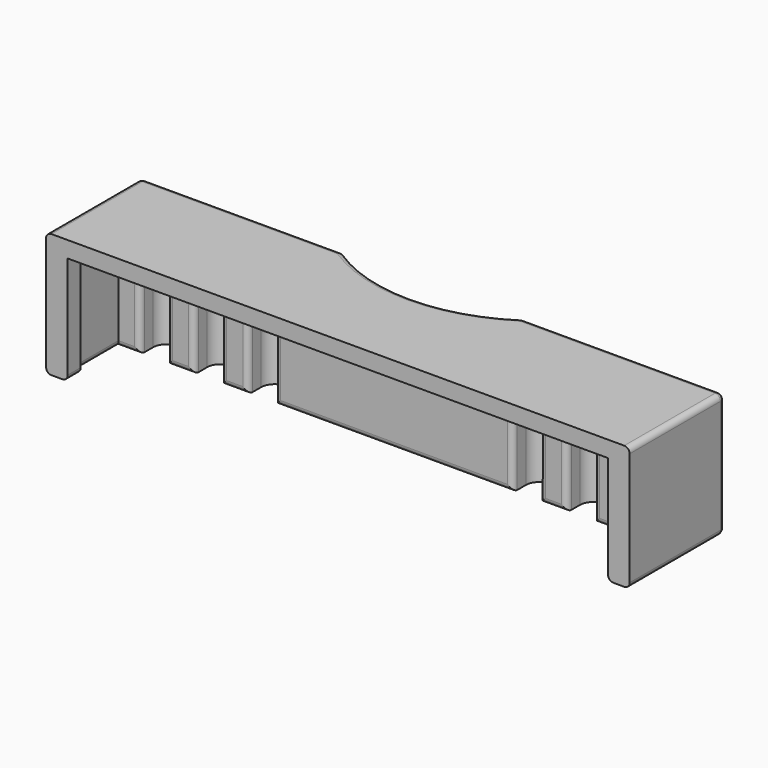
from build123d import *

# Parameters (mm, degrees)
F0_W     = 1
F0_H     = 20
F0_W_2   = 100
F1_DEPTH = 22
F2_DEPTH = 13
F3_DEPTH = 3
F5_DEPTH = 23
F4_W     = 5
F4_H     = 3
F6_DEPTH = 20
F7_R     = 0.9999


# Not quite as in the source:
# - a fillet or chamfer is up to 0.001 mm smaller than in the source, because OpenCascade refuses the exact size
# - a feature names something its author has since deleted; it is built from what else it names


with BuildPart() as f1:
    # F0 (on Front) → F1 (new body)
    with BuildSketch(Plane.XZ):
        Polygon((51, 20), (51, 0), (54, 0), (54, 23), (-54, 23), (-54, 0), (-51, 0), (-51, 20), (-50, 20), (50, 20), align=None)
        with Locations((-50.5, 10)):
            Rectangle(F0_W, F0_H)
        with Locations((0, 10)):
            Rectangle(F0_W_2, F0_H)
        with Locations((50.5, 10)):
            Rectangle(F0_W, F0_H)
    extrude(amount=-F1_DEPTH)

    # F0 (on Front) → F2 (cut)
    with BuildSketch(Plane.XZ):
        with Locations((-50.5, 10)):
            Rectangle(F0_W, F0_H)
        with Locations((0, 10)):
            Rectangle(F0_W_2, F0_H)
        with Locations((50.5, 10)):
            Rectangle(F0_W, F0_H)
    extrude(amount=-F2_DEPTH, mode=Mode.SUBTRACT)

    # F0 (on Front) → F3 (join)
    with BuildSketch(Plane.XZ):
        with Locations((-50.5, 10)):
            Rectangle(F0_W, F0_H)
        with Locations((50.5, 10)):
            Rectangle(F0_W, F0_H)
    extrude(amount=-F3_DEPTH)

    # F4 (on face) → F5 (cut, through all)
    with BuildSketch(Plane(origin=(0, 0, 0), x_dir=(1, 0, 0), z_dir=(0, 0, -1))):
        with BuildLine():
            Line((-16.5831239518, -22), (16.5831239518, -22))
            ThreePointArc((16.5831239518, -22), (0, -17), (-16.5831239518, -22))
        make_face()
    extrude(amount=-F5_DEPTH, mode=Mode.SUBTRACT)

    # F4 (on face) → F6 (cut, through all)
    with BuildSketch(Plane(origin=(0, 0, 0), x_dir=(1, 0, 0), z_dir=(0, 0, -1))):
        with Locations((-44.5, -14.5)):
            Rectangle(F4_W, F4_H)
        with Locations((-34.5, -14.5)):
            Rectangle(F4_W, F4_H)
        with Locations((-24.5, -14.5)):
            Rectangle(F4_W, F4_H)
        with Locations((24.5, -14.5)):
            Rectangle(F4_W, F4_H)
        with Locations((34.5, -14.5)):
            Rectangle(F4_W, F4_H)
        with Locations((44.5, -14.5)):
            Rectangle(F4_W, F4_H)
        with BuildLine():
            Line((-42, -16), (-47, -16))
            ThreePointArc((-47, -16), (-44.5, -18.5), (-42, -16))
        make_face()
        with BuildLine():
            Line((-32, -16), (-37, -16))
            ThreePointArc((-37, -16), (-34.5, -18.5), (-32, -16))
        make_face()
        with BuildLine():
            Line((-22, -16), (-27, -16))
            ThreePointArc((-27, -16), (-24.5, -18.5), (-22, -16))
        make_face()
        with BuildLine():
            ThreePointArc((22, -16), (24.5, -18.5), (27, -16))
            Line((27, -16), (22, -16))
        make_face()
        with BuildLine():
            ThreePointArc((32, -16), (34.5, -18.5), (37, -16))
            Line((37, -16), (32, -16))
        make_face()
        with BuildLine():
            ThreePointArc((42, -16), (44.5, -18.5), (47, -16))
            Line((47, -16), (42, -16))
        make_face()
    extrude(amount=-F6_DEPTH, mode=Mode.SUBTRACT)

    # F7 (radius 1 in the source; OpenCascade refuses exactly that, so slightly less here)
    f7_edges = [f1.edges().sort_by_distance(p)[0] for p in [
        (-54, 22, 11.5),
        (54, 22, 11.5),
        (35.291562, 22, 0),
        (-35.291562, 22, 0),
        (54, 11, 0),
        (-54, 11, 0),
        (-54, 11, 23),
        (-35.291562, 22, 23),
        (35.291562, 22, 23),
        (54, 11, 23),
        (-49, 13, 0),
        (-39.5, 13, 0),
        (-29.5, 13, 0),
        (0, 13, 0),
        (29.5, 13, 0),
        (39.5, 13, 0),
        (49, 13, 0),
        (51, 8, 0),
        (-51, 8, 0),
        (-50, 1.5, 0),
        (50, 1.5, 0),
        (0, 17, 23),
        (0, 17, 0),
        (-47, 13, 10),
        (-42, 13, 10),
        (-37, 13, 10),
        (-32, 13, 10),
        (-27, 13, 10),
        (-22, 13, 10),
        (22, 13, 10),
        (27, 13, 10),
        (32, 13, 10),
        (47, 13, 10),
        (42, 13, 10),
        (37, 13, 10),
        (16.583124, 22, 11.5),
        (-16.583124, 22, 11.5),
    ]]
    fillet(f7_edges, radius=F7_R)


solid = f1.part
